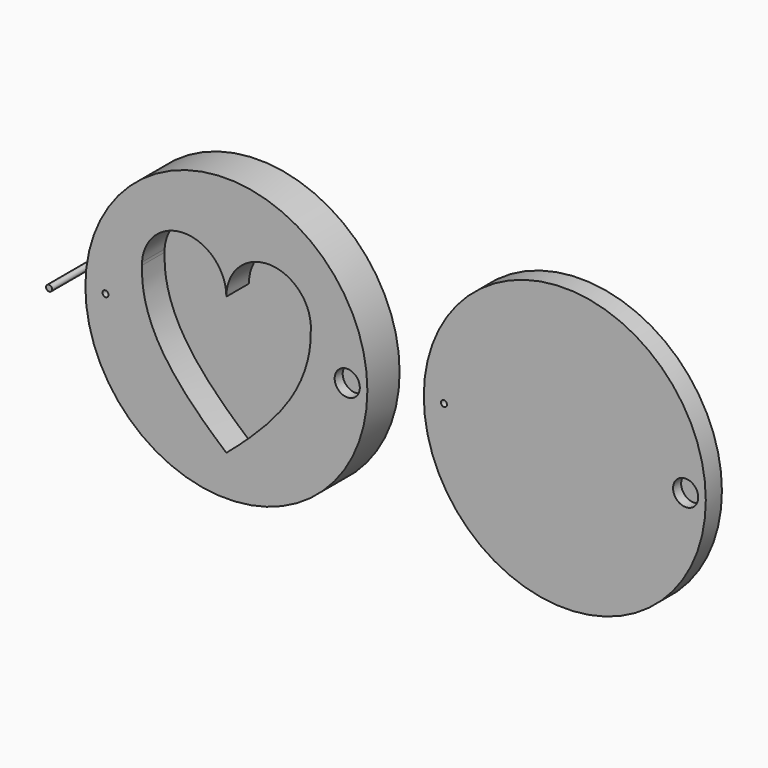
from build123d import *

# Parameters (mm, degrees)
F0_R     = 44.45
F0_R_2   = 0.9525
F0_R_3   = 3.96875
F1_DEPTH = 12.7
F2_DEPTH = 3.81
F3_DEPTH = 9.525
F4_DEPTH = 6.35
F5_DEPTH = 3.175
F6_DEPTH = 19.05


with BuildPart() as f1:
    # F0 (on Front) → F1 (new body)
    with BuildSketch(Plane.XZ):
        Circle(F0_R)
        with BuildLine():
            ThreePointArc((-12.2481151241, 24.8639554142), (-3.5297989426, 20.6200957751), (0, 11.5890437267))
            ThreePointArc((0, 11.5890437267), (3.5297989426, 20.6200957751), (12.2481151241, 24.8639554142))
            add(Edge.make_bspline(
                [(12.2481151241, 24.8639554142), (14.6922572571, 26.4350209104), (22.4074488188, 29.3295793858), (26.2533609705, 19.9457695703), (26.6043971909, 12.5045702251)],
                knots=[0.201568932, 0.201568932, 0.201568932, 0.201568932, 0.3004267747, 0.5168406107, 0.5168406107, 0.5168406107, 0.5168406107], degree=3))
            ThreePointArc((26.6043971909, 12.5045702251), (26.6280240963, 12.0470779435), (26.6359028388, 11.5890437267))
            add(Edge.make_bspline(
                [(26.6359028388, 11.5890437267), (26.6898066873, 9.1110835654), (25.3801041465, -7.941133268), (12.2456271202, -21.2775729597), (0, -31.75)],
                knots=[0.5256708302, 0.5256708302, 0.5256708302, 0.5256708302, 0.5970317864, 1, 1, 1, 1], degree=3))
            add(Edge.make_bspline(
                [(-26.6359028388, 11.5890437267), (-26.6898066873, 9.1110835654), (-25.3801041465, -7.941133268), (-12.2456271202, -21.2775729597), (0, -31.75)],
                knots=[0.5256708302, 0.5256708302, 0.5256708302, 0.5256708302, 0.5970317864, 1, 1, 1, 1], degree=3))
            ThreePointArc((-26.6359028388, 11.5890437267), (-26.6280240963, 12.0470779435), (-26.6043971909, 12.5045702251))
            add(Edge.make_bspline(
                [(-12.2481151241, 24.8639554142), (-14.6922572571, 26.4350209104), (-22.4074488188, 29.3295793858), (-26.2533609705, 19.9457695703), (-26.6043971909, 12.5045702251)],
                knots=[0.201568932, 0.201568932, 0.201568932, 0.201568932, 0.3004267747, 0.5168406107, 0.5168406107, 0.5168406107, 0.5168406107], degree=3))
        make_face(mode=Mode.SUBTRACT)
        with Locations((-38.1, 0)):
            Circle(F0_R_2, mode=Mode.SUBTRACT)
        with Locations((38.1, 0)):
            Circle(F0_R_3, mode=Mode.SUBTRACT)
        with BuildLine():
            ThreePointArc((-26.6043971909, 12.5045702251), (-22.0070242892, 21.6820037817), (-12.2481151241, 24.8639554142))
            add(Edge.make_bspline(
                [(-12.2481151241, 24.8639554142), (-14.6922572571, 26.4350209104), (-22.4074488188, 29.3295793858), (-26.2533609705, 19.9457695703), (-26.6043971909, 12.5045702251)],
                knots=[0.201568932, 0.201568932, 0.201568932, 0.201568932, 0.3004267747, 0.5168406107, 0.5168406107, 0.5168406107, 0.5168406107], degree=3))
        make_face()
        with BuildLine():
            add(Edge.make_bspline(
                [(12.2481151241, 24.8639554142), (14.6922572571, 26.4350209104), (22.4074488188, 29.3295793858), (26.2533609705, 19.9457695703), (26.6043971909, 12.5045702251)],
                knots=[0.201568932, 0.201568932, 0.201568932, 0.201568932, 0.3004267747, 0.5168406107, 0.5168406107, 0.5168406107, 0.5168406107], degree=3))
            ThreePointArc((12.2481151241, 24.8639554142), (22.0070242892, 21.6820037817), (26.6043971909, 12.5045702251))
        make_face()
    extrude(amount=F1_DEPTH)

    # F0 (on Front) → F2 (join)
    with BuildSketch(Plane.XZ):
        with BuildLine():
            add(Edge.make_bspline(
                [(0, 11.5890437267), (-2.1773432855, 15.6990310035), (-7.2645639382, 21.6605879785), (-12.2481151241, 24.8639554142)],
                knots=[0, 0, 0, 0, 0.201568932, 0.201568932, 0.201568932, 0.201568932], degree=3))
            ThreePointArc((0, 11.5890437267), (-3.5297989426, 20.6200957751), (-12.2481151241, 24.8639554142))
        make_face()
        with BuildLine():
            add(Edge.make_bspline(
                [(0, 11.5890437267), (2.1773432855, 15.6990310035), (7.2645639382, 21.6605879785), (12.2481151241, 24.8639554142)],
                knots=[0, 0, 0, 0, 0.201568932, 0.201568932, 0.201568932, 0.201568932], degree=3))
            add(Edge.make_bspline(
                [(0, 11.5890437267), (-2.1773432855, 15.6990310035), (-7.2645639382, 21.6605879785), (-12.2481151241, 24.8639554142)],
                knots=[0, 0, 0, 0, 0.201568932, 0.201568932, 0.201568932, 0.201568932], degree=3))
            ThreePointArc((-12.2481151241, 24.8639554142), (-22.0070242892, 21.6820037817), (-26.6043971909, 12.5045702251))
            add(Edge.make_bspline(
                [(-26.6043971909, 12.5045702251), (-26.6187203366, 12.2009508949), (-26.6292327654, 11.8956670321), (-26.6359028388, 11.5890437267)],
                knots=[0.5168406107, 0.5168406107, 0.5168406107, 0.5168406107, 0.5256708302, 0.5256708302, 0.5256708302, 0.5256708302], degree=3))
            add(Edge.make_bspline(
                [(-26.6359028388, 11.5890437267), (-26.6898066873, 9.1110835654), (-25.3801041465, -7.941133268), (-12.2456271202, -21.2775729597), (0, -31.75)],
                knots=[0.5256708302, 0.5256708302, 0.5256708302, 0.5256708302, 0.5970317864, 1, 1, 1, 1], degree=3))
            add(Edge.make_bspline(
                [(26.6359028388, 11.5890437267), (26.6898066873, 9.1110835654), (25.3801041465, -7.941133268), (12.2456271202, -21.2775729597), (0, -31.75)],
                knots=[0.5256708302, 0.5256708302, 0.5256708302, 0.5256708302, 0.5970317864, 1, 1, 1, 1], degree=3))
            add(Edge.make_bspline(
                [(26.6043971909, 12.5045702251), (26.6187203366, 12.2009508949), (26.6292327654, 11.8956670321), (26.6359028388, 11.5890437267)],
                knots=[0.5168406107, 0.5168406107, 0.5168406107, 0.5168406107, 0.5256708302, 0.5256708302, 0.5256708302, 0.5256708302], degree=3))
            ThreePointArc((26.6043971909, 12.5045702251), (22.0070242892, 21.6820037817), (12.2481151241, 24.8639554142))
        make_face()
        with BuildLine():
            ThreePointArc((12.2481151241, 24.8639554142), (3.5297989426, 20.6200957751), (0, 11.5890437267))
            add(Edge.make_bspline(
                [(0, 11.5890437267), (2.1773432855, 15.6990310035), (7.2645639382, 21.6605879785), (12.2481151241, 24.8639554142)],
                knots=[0, 0, 0, 0, 0.201568932, 0.201568932, 0.201568932, 0.201568932], degree=3))
        make_face()
        with BuildLine():
            ThreePointArc((-26.6043971909, 12.5045702251), (-22.0070242892, 21.6820037817), (-12.2481151241, 24.8639554142))
            add(Edge.make_bspline(
                [(-12.2481151241, 24.8639554142), (-14.6922572571, 26.4350209104), (-22.4074488188, 29.3295793858), (-26.2533609705, 19.9457695703), (-26.6043971909, 12.5045702251)],
                knots=[0.201568932, 0.201568932, 0.201568932, 0.201568932, 0.3004267747, 0.5168406107, 0.5168406107, 0.5168406107, 0.5168406107], degree=3))
        make_face()
        with BuildLine():
            add(Edge.make_bspline(
                [(12.2481151241, 24.8639554142), (14.6922572571, 26.4350209104), (22.4074488188, 29.3295793858), (26.2533609705, 19.9457695703), (26.6043971909, 12.5045702251)],
                knots=[0.201568932, 0.201568932, 0.201568932, 0.201568932, 0.3004267747, 0.5168406107, 0.5168406107, 0.5168406107, 0.5168406107], degree=3))
            ThreePointArc((12.2481151241, 24.8639554142), (22.0070242892, 21.6820037817), (26.6043971909, 12.5045702251))
        make_face()
        with BuildLine():
            add(Edge.make_bspline(
                [(-26.6043971909, 12.5045702251), (-26.6187203366, 12.2009508949), (-26.6292327654, 11.8956670321), (-26.6359028388, 11.5890437267)],
                knots=[0.5168406107, 0.5168406107, 0.5168406107, 0.5168406107, 0.5256708302, 0.5256708302, 0.5256708302, 0.5256708302], degree=3))
            ThreePointArc((-26.6043971909, 12.5045702251), (-26.6280240963, 12.0470779435), (-26.6359028388, 11.5890437267))
        make_face()
        with BuildLine():
            ThreePointArc((26.6359028388, 11.5890437267), (26.6280240963, 12.0470779435), (26.6043971909, 12.5045702251))
            add(Edge.make_bspline(
                [(26.6043971909, 12.5045702251), (26.6187203366, 12.2009508949), (26.6292327654, 11.8956670321), (26.6359028388, 11.5890437267)],
                knots=[0.5168406107, 0.5168406107, 0.5168406107, 0.5168406107, 0.5256708302, 0.5256708302, 0.5256708302, 0.5256708302], degree=3))
        make_face()
    extrude(amount=F2_DEPTH)

    # F0 (on Front) → F3 (join)
    with BuildSketch(Plane.XZ):
        with Locations((38.1, 0)):
            Circle(F0_R_3)
    extrude(amount=F3_DEPTH)


with BuildPart() as f4:
    # F0 (on Front) → F4 (new body)
    with BuildSketch(Plane.XZ):
        with Locations((101.6, 0)):
            Circle(F0_R)
        with Locations((63.5, 0)):
            Circle(F0_R_2, mode=Mode.SUBTRACT)
        with Locations((139.7, 0)):
            Circle(F0_R_3, mode=Mode.SUBTRACT)
    extrude(amount=F4_DEPTH)

    # F0 (on Front) → F5 (join)
    with BuildSketch(Plane.XZ):
        with Locations((139.7, 0)):
            Circle(F0_R_3)
    extrude(amount=F5_DEPTH)


with BuildPart() as f6:
    # F0 (on Front) → F6 (new body)
    with BuildSketch(Plane.XZ):
        with Locations((-50.8, 0)):
            Circle(F0_R_2)
    extrude(amount=F6_DEPTH)


solid = Compound([f1.part, f4.part, f6.part])
